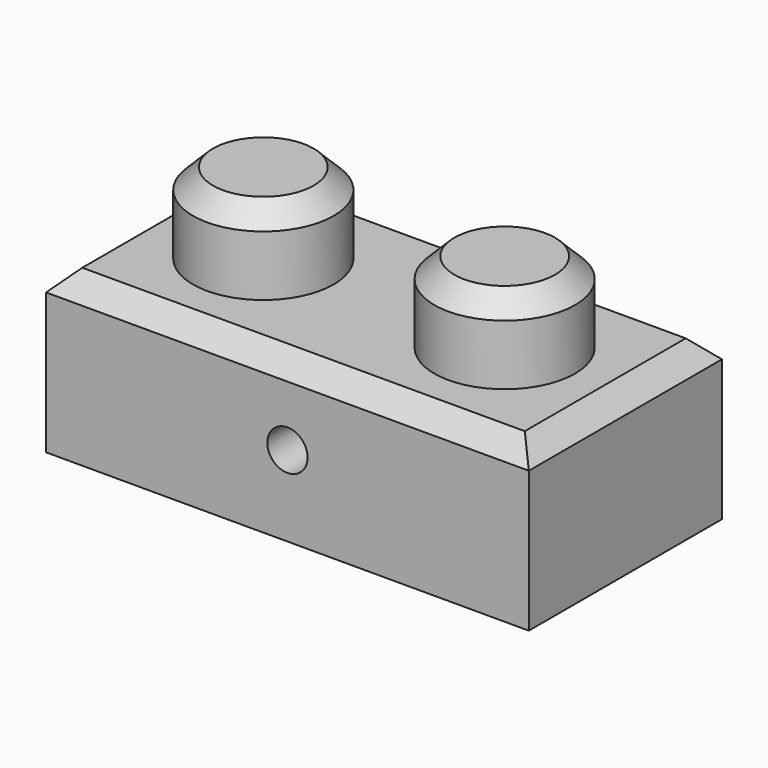
from build123d import *

# Parameters (mm, degrees)
F0_W          = 76.2
F0_H          = 38.1
F1_DEPTH      = 25.4
F2_R          = 11.1125
F3_DEPTH      = 12.7
F4_R          = 3.175
F5_DEPTH      = 38.101
F5_DEPTH_BACK = 139
F6_SIZE       = 3.175


# Not quite as in the source:
# - an extrude ends at something that could not be found from the text; its depth is read off the source's solid


with BuildPart() as f1:
    # F0 (on Top) → F1 (new body)
    with BuildSketch(Plane.XY):
        with Locations((38.1, -19.05)):
            Rectangle(F0_W, F0_H)
    extrude(amount=F1_DEPTH)

    # F2 (on face) → F3 (join)
    with BuildSketch(Plane.XY.offset(25.4)):
        with Locations((19.05, -19.05)):
            Circle(F2_R)
        with Locations((57.15, -19.05)):
            Circle(F2_R)
    extrude(amount=F3_DEPTH)

    # F4 (on face) → F5 (cut, two sides)
    with BuildSketch(Plane.XZ.offset(38.1)) as f5_sk:
        with Locations((38.1, 12.7)):
            Circle(F4_R)
    extrude(amount=-F5_DEPTH, mode=Mode.SUBTRACT)
    extrude(f5_sk.sketch, amount=F5_DEPTH_BACK, mode=Mode.SUBTRACT)

    # F6
    f6_edges = [f1.edges().sort_by_distance(p)[0] for p in [
        (46.0375, -19.05, 38.1),
        (7.9375, -19.05, 38.1),
        (38.1, -38.1, 25.4),
        (76.2, -19.05, 25.4),
        (38.1, 0, 25.4),
        (0, -19.05, 25.4),
    ]]
    chamfer(f6_edges, length=F6_SIZE)


solid = f1.part
